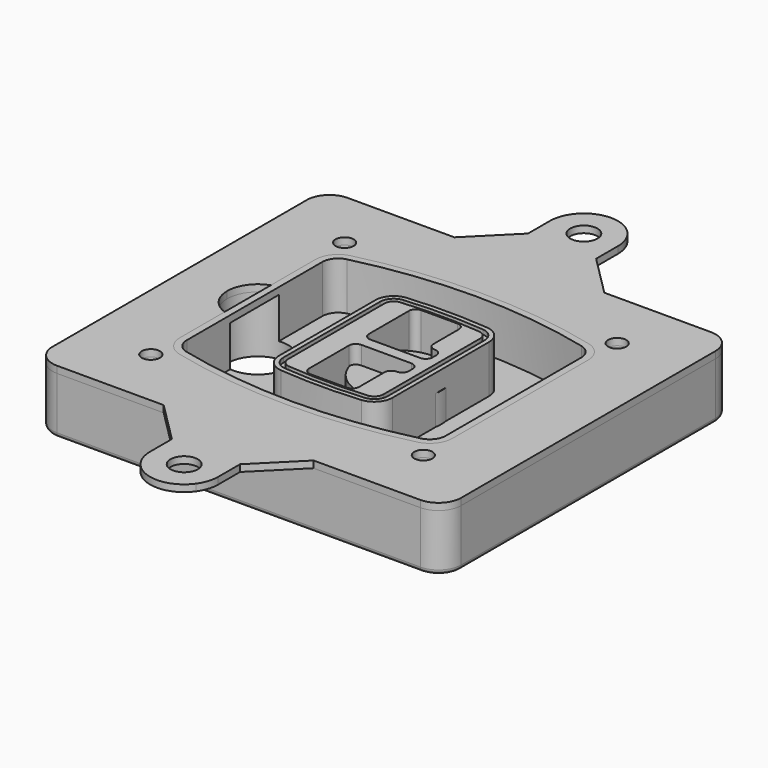
from build123d import *

# Parameters (mm, degrees)
F0_R      = 4
F1_DEPTH  = 25
F2_DEPTH  = 3
F3_DEPTH  = 18
F5_DEPTH  = 21
F6_DEPTH  = 2
F8_DEPTH  = 20
F9_DEPTH  = 16
F10_DEPTH = 25
F7_R      = 6
F7_R_2    = 4
F11_DEPTH = 6
F13_DEPTH = 9
F15_R     = 2
F16_R     = 6
F16_R_2   = 4
F17_DEPTH = 3


# Not quite as in the source:
# - a feature of the source that left no trace in its solid (it failed there, or was rolled back) is left out
# - a feature names something its author has since deleted; it is built from what else it names


with BuildPart() as f1:
    # F0 (on Top) → F1 (new body)
    with BuildSketch(Plane.XY):
        with BuildLine():
            ThreePointArc((-90, -70), (-87.0710678119, -77.0710678119), (-80, -80))
            Line((-80, -80), (80, -80))
            ThreePointArc((80, -80), (87.0710678119, -77.0710678119), (90, -70))
            Line((90, -70), (90, 70))
            ThreePointArc((90, 70), (87.0710678119, 77.0710678119), (80, 80))
            Line((80, 80), (-80, 80))
            ThreePointArc((-80, 80), (-87.0710678119, 77.0710678119), (-90, 70))
            Line((-90, 70), (-90, -70))
        make_face()
        with Locations((-60, -53.3333333333)):
            Circle(F0_R, mode=Mode.SUBTRACT)
        with Locations((60, -53.3333333333)):
            Circle(F0_R, mode=Mode.SUBTRACT)
        with Locations((-60, 53.3333333333)):
            Circle(F0_R, mode=Mode.SUBTRACT)
        with BuildLine():
            ThreePointArc((-64, 37.2990447398), (-61.0143011354, 45.9411029726), (-53.3306899286, 50.8970778549))
            ThreePointArc((-53.3306899286, 50.8970778549), (0, 57.3333333333), (53.3306899286, 50.8970778549))
            ThreePointArc((53.3306899286, 50.8970778549), (61.0143011354, 45.9411029726), (64, 37.2990447398))
            Line((64, 37.2990447398), (64, -37.2990447398))
            ThreePointArc((64, -37.2990447398), (61.0143011354, -45.9411029726), (53.3306899286, -50.8970778549))
            ThreePointArc((53.3306899286, -50.8970778549), (0, -57.3333333333), (-53.3306899286, -50.8970778549))
            ThreePointArc((-53.3306899286, -50.8970778549), (-61.0143011354, -45.9411029726), (-64, -37.2990447398))
            Line((-64, -37.2990447398), (-64, 37.2990447398))
        make_face(mode=Mode.SUBTRACT)
        with Locations((60, 53.3333333333)):
            Circle(F0_R, mode=Mode.SUBTRACT)
        with BuildLine():
            ThreePointArc((53.3306899286, 50.8970778549), (0, 57.3333333333), (-53.3306899286, 50.8970778549))
            ThreePointArc((-53.3306899286, 50.8970778549), (-61.0143011354, 45.9411029726), (-64, 37.2990447398))
            Line((-64, 37.2990447398), (-64, -37.2990447398))
            ThreePointArc((-64, -37.2990447398), (-61.0143011354, -45.9411029726), (-53.3306899286, -50.8970778549))
            ThreePointArc((-53.3306899286, -50.8970778549), (0, -57.3333333333), (53.3306899286, -50.8970778549))
            ThreePointArc((53.3306899286, -50.8970778549), (61.0143011354, -45.9411029726), (64, -37.2990447398))
            Line((64, -37.2990447398), (64, 37.2990447398))
            ThreePointArc((64, 37.2990447398), (61.0143011354, 45.9411029726), (53.3306899286, 50.8970778549))
        make_face()
        with BuildLine():
            Line((-60, -37.2990447398), (-60, 37.2990447398))
            ThreePointArc((-60, 37.2990447398), (-57.8673579538, 43.4719434775), (-52.3790642347, 47.0119255363))
            ThreePointArc((-52.3790642347, 47.0119255363), (0, 53.3333333333), (52.3790642347, 47.0119255363))
            ThreePointArc((52.3790642347, 47.0119255363), (57.8673579538, 43.4719434775), (60, 37.2990447398))
            Line((60, 37.2990447398), (60, -37.2990447398))
            ThreePointArc((60, -37.2990447398), (57.8673579538, -43.4719434775), (52.3790642347, -47.0119255363))
            ThreePointArc((52.3790642347, -47.0119255363), (0, -53.3333333333), (-52.3790642347, -47.0119255363))
            ThreePointArc((-52.3790642347, -47.0119255363), (-57.8673579538, -43.4719434775), (-60, -37.2990447398))
        make_face(mode=Mode.SUBTRACT)
        with BuildLine():
            ThreePointArc((-52.3790642347, 47.0119255363), (-57.8673579538, 43.4719434775), (-60, 37.2990447398))
            Line((-60, 37.2990447398), (-60, -37.2990447398))
            ThreePointArc((-60, -37.2990447398), (-57.8673579538, -43.4719434775), (-52.3790642347, -47.0119255363))
            ThreePointArc((-52.3790642347, -47.0119255363), (0, -53.3333333333), (52.3790642347, -47.0119255363))
            ThreePointArc((52.3790642347, -47.0119255363), (57.8673579538, -43.4719434775), (60, -37.2990447398))
            Line((60, -37.2990447398), (60, 37.2990447398))
            ThreePointArc((60, 37.2990447398), (57.8673579538, 43.4719434775), (52.3790642347, 47.0119255363))
            ThreePointArc((52.3790642347, 47.0119255363), (0, 53.3333333333), (-52.3790642347, 47.0119255363))
        make_face()
        with BuildLine():
            ThreePointArc((51.6653449643, 44.0980612973), (55.5071505677, 41.6200738562), (57, 37.2990447398))
            Line((57, 37.2990447398), (57, -37.2990447398))
            ThreePointArc((57, -37.2990447398), (55.5071505677, -41.6200738562), (51.6653449643, -44.0980612973))
            ThreePointArc((51.6653449643, -44.0980612973), (0, -50.3333333333), (-51.6653449643, -44.0980612973))
            ThreePointArc((-51.6653449643, -44.0980612973), (-55.5071505677, -41.6200738562), (-57, -37.2990447398))
            Line((-57, -37.2990447398), (-57, 37.2990447398))
            ThreePointArc((-57, 37.2990447398), (-55.5071505677, 41.6200738562), (-51.6653449643, 44.0980612973))
            ThreePointArc((-51.6653449643, 44.0980612973), (0, 50.3333333333), (51.6653449643, 44.0980612973))
        make_face(mode=Mode.SUBTRACT)
        with BuildLine():
            Line((57, -37.2990447398), (57, 37.2990447398))
            ThreePointArc((57, 37.2990447398), (55.5071505677, 41.6200738562), (51.6653449643, 44.0980612973))
            ThreePointArc((51.6653449643, 44.0980612973), (0, 50.3333333333), (-51.6653449643, 44.0980612973))
            ThreePointArc((-51.6653449643, 44.0980612973), (-55.5071505677, 41.6200738562), (-57, 37.2990447398))
            Line((-57, 37.2990447398), (-57, -37.2990447398))
            ThreePointArc((-57, -37.2990447398), (-55.5071505677, -41.6200738562), (-51.6653449643, -44.0980612973))
            ThreePointArc((-51.6653449643, -44.0980612973), (0, -50.3333333333), (51.6653449643, -44.0980612973))
            ThreePointArc((51.6653449643, -44.0980612973), (55.5071505677, -41.6200738562), (57, -37.2990447398))
        make_face()
    extrude(amount=-F1_DEPTH)

    # F0 (on Top) → F2 (join)
    with BuildSketch(Plane.XY):
        with BuildLine():
            ThreePointArc((-52.3790642347, 47.0119255363), (-57.8673579538, 43.4719434775), (-60, 37.2990447398))
            Line((-60, 37.2990447398), (-60, -37.2990447398))
            ThreePointArc((-60, -37.2990447398), (-57.8673579538, -43.4719434775), (-52.3790642347, -47.0119255363))
            ThreePointArc((-52.3790642347, -47.0119255363), (0, -53.3333333333), (52.3790642347, -47.0119255363))
            ThreePointArc((52.3790642347, -47.0119255363), (57.8673579538, -43.4719434775), (60, -37.2990447398))
            Line((60, -37.2990447398), (60, 37.2990447398))
            ThreePointArc((60, 37.2990447398), (57.8673579538, 43.4719434775), (52.3790642347, 47.0119255363))
            ThreePointArc((52.3790642347, 47.0119255363), (0, 53.3333333333), (-52.3790642347, 47.0119255363))
        make_face()
        with BuildLine():
            ThreePointArc((51.6653449643, 44.0980612973), (55.5071505677, 41.6200738562), (57, 37.2990447398))
            Line((57, 37.2990447398), (57, -37.2990447398))
            ThreePointArc((57, -37.2990447398), (55.5071505677, -41.6200738562), (51.6653449643, -44.0980612973))
            ThreePointArc((51.6653449643, -44.0980612973), (0, -50.3333333333), (-51.6653449643, -44.0980612973))
            ThreePointArc((-51.6653449643, -44.0980612973), (-55.5071505677, -41.6200738562), (-57, -37.2990447398))
            Line((-57, -37.2990447398), (-57, 37.2990447398))
            ThreePointArc((-57, 37.2990447398), (-55.5071505677, 41.6200738562), (-51.6653449643, 44.0980612973))
            ThreePointArc((-51.6653449643, 44.0980612973), (0, 50.3333333333), (51.6653449643, 44.0980612973))
        make_face(mode=Mode.SUBTRACT)
    extrude(amount=F2_DEPTH)

    # F0 (on Top) → F3 (cut)
    with BuildSketch(Plane.XY):
        with BuildLine():
            Line((57, -37.2990447398), (57, 37.2990447398))
            ThreePointArc((57, 37.2990447398), (55.5071505677, 41.6200738562), (51.6653449643, 44.0980612973))
            ThreePointArc((51.6653449643, 44.0980612973), (0, 50.3333333333), (-51.6653449643, 44.0980612973))
            ThreePointArc((-51.6653449643, 44.0980612973), (-55.5071505677, 41.6200738562), (-57, 37.2990447398))
            Line((-57, 37.2990447398), (-57, -37.2990447398))
            ThreePointArc((-57, -37.2990447398), (-55.5071505677, -41.6200738562), (-51.6653449643, -44.0980612973))
            ThreePointArc((-51.6653449643, -44.0980612973), (0, -50.3333333333), (51.6653449643, -44.0980612973))
            ThreePointArc((51.6653449643, -44.0980612973), (55.5071505677, -41.6200738562), (57, -37.2990447398))
        make_face()
    extrude(amount=-F3_DEPTH, mode=Mode.SUBTRACT)

    # F4 (on face) → F5 (join, through all)
    with BuildSketch(Plane.XY.offset(3)):
        with BuildLine():
            ThreePointArc((-25, -26.587695628), (-22.8992979869, -31.9912392117), (-17.7004291845, -34.5569740744))
            ThreePointArc((-17.7004291845, -34.5569740744), (0, -35.3333333333), (17.7004291845, -34.5569740744))
            ThreePointArc((17.7004291845, -34.5569740744), (22.8992979869, -31.9912392117), (25, -26.587695628))
            Line((25, -26.587695628), (25, 26.587695628))
            ThreePointArc((25, 26.587695628), (22.8992979869, 31.9912392117), (17.7004291845, 34.5569740744))
            ThreePointArc((17.7004291845, 34.5569740744), (0, 35.3333333333), (-17.7004291845, 34.5569740744))
            ThreePointArc((-17.7004291845, 34.5569740744), (-22.8992979869, 31.9912392117), (-25, 26.587695628))
            Line((-25, 26.587695628), (-25, -26.587695628))
        make_face()
        with BuildLine():
            ThreePointArc((17.5253218884, 32.5646544628), (21.4244734902, 30.6403533158), (23, 26.587695628))
            Line((23, 26.587695628), (23, -26.587695628))
            ThreePointArc((23, -26.587695628), (21.4244734902, -30.6403533158), (17.5253218884, -32.5646544628))
            ThreePointArc((17.5253218884, -32.5646544628), (0, -33.3333333333), (-17.5253218884, -32.5646544628))
            ThreePointArc((-17.5253218884, -32.5646544628), (-21.4244734902, -30.6403533158), (-23, -26.587695628))
            Line((-23, -26.587695628), (-23, 26.587695628))
            ThreePointArc((-23, 26.587695628), (-21.4244734902, 30.6403533158), (-17.5253218884, 32.5646544628))
            ThreePointArc((-17.5253218884, 32.5646544628), (0, 33.3333333333), (17.5253218884, 32.5646544628))
        make_face(mode=Mode.SUBTRACT)
        with BuildLine():
            Line((23, -26.587695628), (23, 26.587695628))
            ThreePointArc((23, 26.587695628), (21.4244734902, 30.6403533158), (17.5253218884, 32.5646544628))
            ThreePointArc((17.5253218884, 32.5646544628), (0, 33.3333333333), (-17.5253218884, 32.5646544628))
            ThreePointArc((-17.5253218884, 32.5646544628), (-21.4244734902, 30.6403533158), (-23, 26.587695628))
            Line((-23, 26.587695628), (-23, -26.587695628))
            ThreePointArc((-23, -26.587695628), (-21.4244734902, -30.6403533158), (-17.5253218884, -32.5646544628))
            ThreePointArc((-17.5253218884, -32.5646544628), (0, -33.3333333333), (17.5253218884, -32.5646544628))
            ThreePointArc((17.5253218884, -32.5646544628), (21.4244734902, -30.6403533158), (23, -26.587695628))
        make_face()
        with BuildLine():
            ThreePointArc((17.3502145923, 30.5723348512), (19.9496489934, 29.2894674198), (21, 26.587695628))
            Line((21, 26.587695628), (21, -26.587695628))
            ThreePointArc((21, -26.587695628), (19.9496489934, -29.2894674198), (17.3502145923, -30.5723348512))
            ThreePointArc((17.3502145923, -30.5723348512), (0, -31.3333333333), (-17.3502145923, -30.5723348512))
            ThreePointArc((-17.3502145923, -30.5723348512), (-19.9496489934, -29.2894674198), (-21, -26.587695628))
            Line((-21, -26.587695628), (-21, 26.587695628))
            ThreePointArc((-21, 26.587695628), (-19.9496489934, 29.2894674198), (-17.3502145923, 30.5723348512))
            ThreePointArc((-17.3502145923, 30.5723348512), (0, 31.3333333333), (17.3502145923, 30.5723348512))
        make_face(mode=Mode.SUBTRACT)
        with BuildLine():
            Line((21, -26.587695628), (21, 26.587695628))
            ThreePointArc((21, 26.587695628), (19.9496489934, 29.2894674198), (17.3502145923, 30.5723348512))
            ThreePointArc((17.3502145923, 30.5723348512), (0, 31.3333333333), (-17.3502145923, 30.5723348512))
            ThreePointArc((-17.3502145923, 30.5723348512), (-19.9496489934, 29.2894674198), (-21, 26.587695628))
            Line((-21, 26.587695628), (-21, -26.587695628))
            ThreePointArc((-21, -26.587695628), (-19.9496489934, -29.2894674198), (-17.3502145923, -30.5723348512))
            ThreePointArc((-17.3502145923, -30.5723348512), (0, -31.3333333333), (17.3502145923, -30.5723348512))
            ThreePointArc((17.3502145923, -30.5723348512), (19.9496489934, -29.2894674198), (21, -26.587695628))
        make_face()
        with BuildLine():
            Line((-8, -2.5), (14, -2.5))
            ThreePointArc((14, -2.5), (16.1213203436, -3.3786796564), (17, -5.5))
            Line((17, -5.5), (17, -7.5))
            ThreePointArc((17, -7.5), (16.1213203436, -9.6213203436), (14, -10.5))
            ThreePointArc((14, -10.5), (11.8786796564, -11.3786796564), (11, -13.5))
            Line((11, -13.5), (11, -27.5))
            ThreePointArc((11, -27.5), (10.1213203436, -29.6213203436), (8, -30.5))
            Line((8, -30.5), (-8, -30.5))
            ThreePointArc((-8, -30.5), (-10.1213203436, -29.6213203436), (-11, -27.5))
            Line((-11, -27.5), (-11, -5.5))
            ThreePointArc((-11, -5.5), (-10.1213203436, -3.3786796564), (-8, -2.5))
        make_face(mode=Mode.SUBTRACT)
        with BuildLine():
            ThreePointArc((-8, 2.5), (-10.1213203436, 3.3786796564), (-11, 5.5))
            Line((-11, 5.5), (-11, 27.5))
            ThreePointArc((-11, 27.5), (-10.1213203436, 29.6213203436), (-8, 30.5))
            Line((-8, 30.5), (8, 30.5))
            ThreePointArc((8, 30.5), (10.1213203436, 29.6213203436), (11, 27.5))
            Line((11, 27.5), (11, 13.5))
            ThreePointArc((11, 13.5), (11.8786796564, 11.3786796564), (14, 10.5))
            ThreePointArc((14, 10.5), (16.1213203436, 9.6213203436), (17, 7.5))
            Line((17, 7.5), (17, 5.5))
            ThreePointArc((17, 5.5), (16.1213203436, 3.3786796564), (14, 2.5))
            Line((14, 2.5), (-8, 2.5))
        make_face(mode=Mode.SUBTRACT)
    extrude(amount=-F5_DEPTH)

    # F4 (on face) → F6 (cut)
    with BuildSketch(Plane.XY.offset(3)):
        with BuildLine():
            Line((23, -26.587695628), (23, 26.587695628))
            ThreePointArc((23, 26.587695628), (21.4244734902, 30.6403533158), (17.5253218884, 32.5646544628))
            ThreePointArc((17.5253218884, 32.5646544628), (0, 33.3333333333), (-17.5253218884, 32.5646544628))
            ThreePointArc((-17.5253218884, 32.5646544628), (-21.4244734902, 30.6403533158), (-23, 26.587695628))
            Line((-23, 26.587695628), (-23, -26.587695628))
            ThreePointArc((-23, -26.587695628), (-21.4244734902, -30.6403533158), (-17.5253218884, -32.5646544628))
            ThreePointArc((-17.5253218884, -32.5646544628), (0, -33.3333333333), (17.5253218884, -32.5646544628))
            ThreePointArc((17.5253218884, -32.5646544628), (21.4244734902, -30.6403533158), (23, -26.587695628))
        make_face()
        with BuildLine():
            ThreePointArc((17.3502145923, 30.5723348512), (19.9496489934, 29.2894674198), (21, 26.587695628))
            Line((21, 26.587695628), (21, -26.587695628))
            ThreePointArc((21, -26.587695628), (19.9496489934, -29.2894674198), (17.3502145923, -30.5723348512))
            ThreePointArc((17.3502145923, -30.5723348512), (0, -31.3333333333), (-17.3502145923, -30.5723348512))
            ThreePointArc((-17.3502145923, -30.5723348512), (-19.9496489934, -29.2894674198), (-21, -26.587695628))
            Line((-21, -26.587695628), (-21, 26.587695628))
            ThreePointArc((-21, 26.587695628), (-19.9496489934, 29.2894674198), (-17.3502145923, 30.5723348512))
            ThreePointArc((-17.3502145923, 30.5723348512), (0, 31.3333333333), (17.3502145923, 30.5723348512))
        make_face(mode=Mode.SUBTRACT)
    extrude(amount=-F6_DEPTH, mode=Mode.SUBTRACT)

    # F7 (on face) → F8 (join)
    with BuildSketch(Plane(origin=(0, 0, -25), x_dir=(1, 0, 0), z_dir=(0, 0, -1))):
        with BuildLine():
            ThreePointArc((-6.71157564, 0), (6.7567035675, 13.4682792075), (20.224982775, 0))
            Line((20.224982775, 0), (25.224982775, 0))
            ThreePointArc((25.224982775, 0), (6.7567035675, 18.4682792075), (-11.71157564, 0))
            Line((-11.71157564, 0), (-6.71157564, 0))
        make_face()
        with BuildLine():
            Line((-6.71157564, 0), (20.224982775, 0))
            ThreePointArc((20.224982775, 0), (6.7567035675, 13.4682792075), (-6.71157564, 0))
        make_face()
        with BuildLine():
            ThreePointArc((-6.71157564, 0), (6.7567035675, -13.4682792075), (20.224982775, 0))
            Line((20.224982775, 0), (-6.71157564, 0))
        make_face()
        with BuildLine():
            Line((25.224982775, 0), (20.224982775, 0))
            ThreePointArc((20.224982775, 0), (6.7567035675, -13.4682792075), (-6.71157564, 0))
            Line((-6.71157564, 0), (-11.71157564, 0))
            ThreePointArc((-11.71157564, 0), (6.7567035675, -18.4682792075), (25.224982775, 0))
        make_face()
    extrude(amount=-F8_DEPTH)

    # F7 (on face) → F9 (cut)
    with BuildSketch(Plane(origin=(0, 0, -25), x_dir=(1, 0, 0), z_dir=(0, 0, -1))):
        with BuildLine():
            Line((-6.71157564, 0), (20.224982775, 0))
            ThreePointArc((20.224982775, 0), (6.7567035675, 13.4682792075), (-6.71157564, 0))
        make_face()
        with BuildLine():
            ThreePointArc((-6.71157564, 0), (6.7567035675, -13.4682792075), (20.224982775, 0))
            Line((20.224982775, 0), (-6.71157564, 0))
        make_face()
    extrude(amount=-F9_DEPTH, mode=Mode.SUBTRACT)

    # F7 (on face) → F10 (cut)
    with BuildSketch(Plane(origin=(0, 0, -25), x_dir=(1, 0, 0), z_dir=(0, 0, -1))):
        with BuildLine():
            Line((-69.0318229325, 0), (-42.0952645175, 0))
            ThreePointArc((-42.0952645175, 0), (-55.563543725, 13.4682792075), (-69.0318229325, 0))
        make_face()
        with BuildLine():
            ThreePointArc((-69.0318229325, 0), (-55.563543725, -13.4682792075), (-42.0952645175, 0))
            Line((-42.0952645175, 0), (-69.0318229325, 0))
        make_face()
    extrude(amount=-F10_DEPTH, mode=Mode.SUBTRACT)

    # F7 (on face) → F11 (cut)
    with BuildSketch(Plane(origin=(0, 0, -25), x_dir=(1, 0, 0), z_dir=(0, 0, -1))):
        with Locations((60, -53.3333333333)):
            Circle(F7_R)
        with Locations((60, -53.3333333333)):
            Circle(F7_R_2, mode=Mode.SUBTRACT)
        with Locations((-60, -53.3333333333)):
            Circle(F7_R)
        with Locations((-60, -53.3333333333)):
            Circle(F7_R_2, mode=Mode.SUBTRACT)
        with Locations((-60, 53.3333333333)):
            Circle(F7_R)
        with Locations((-60, 53.3333333333)):
            Circle(F7_R_2, mode=Mode.SUBTRACT)
        with Locations((60, 53.3333333333)):
            Circle(F7_R)
        with Locations((60, 53.3333333333)):
            Circle(F7_R_2, mode=Mode.SUBTRACT)
    extrude(amount=-F11_DEPTH, mode=Mode.SUBTRACT)

    # F12 (on face) → F13 (cut, through all)
    with BuildSketch(Plane(origin=(0, 0, -9), x_dir=(1, 0, 0), z_dir=(0, 0, -1))):
        with BuildLine():
            ThreePointArc((20.224982775, 0), (20.1663399806, 1.2554664788), (19.9909222755, 2.5))
            Line((19.9909222755, 2.5), (14, 2.5))
            ThreePointArc((14, 2.5), (16.1213203436, 3.3786796564), (17, 5.5))
            Line((17, 5.5), (17, 7.5))
            ThreePointArc((17, 7.5), (16.1213203436, 9.6213203436), (14, 10.5))
            ThreePointArc((14, 10.5), (12.1627255951, 11.1284134507), (11.0951631559, 12.750384826))
            ThreePointArc((11.0951631559, 12.750384826), (11.0476113807, 12.7664660322), (11, 12.7823698976))
            Line((11, 12.7823698976), (11, -12.7823698976))
            ThreePointArc((11, -12.7823698976), (11.0476113807, -12.7664660322), (11.0951631559, -12.750384826))
            ThreePointArc((11.0951631559, -12.750384826), (12.1627255951, -11.1284134507), (14, -10.5))
            ThreePointArc((14, -10.5), (16.1213203436, -9.6213203436), (17, -7.5))
            Line((17, -7.5), (17, -5.5))
            ThreePointArc((17, -5.5), (16.1213203436, -3.3786796564), (14, -2.5))
            Line((14, -2.5), (19.9909222755, -2.5))
            ThreePointArc((19.9909222755, -2.5), (20.1663399806, -1.2554664788), (20.224982775, 0))
        make_face()
    extrude(amount=F13_DEPTH, mode=Mode.SUBTRACT)

    # F15
    f15_edges = [f1.edges().sort_by_distance(p)[0] for p in [
        (0, -80, -25),
        (-87.071068, -77.071068, -25),
        (-90, 0, -25),
        (-87.071068, 77.071068, -25),
        (87.071068, -77.071068, -25),
        (0, 80, -25),
        (90, 0, -25),
        (87.071068, 77.071068, -25),
    ]]
    fillet(f15_edges, radius=F15_R)


with BuildPart() as f17:
    # F16 (on face) → F17 (new body, through all)
    with BuildSketch(Plane.XY):
        with BuildLine():
            ThreePointArc((15, 110), (14.2918775795, 114.5543644179), (12.2343686332, 118.6787224952))
            ThreePointArc((12.2343686332, 118.6787224952), (0, 125), (-12.2343686332, 118.6787224952))
            ThreePointArc((-12.2343686332, 118.6787224952), (-14.2918775795, 114.5543644179), (-15, 110))
            Line((-15, 110), (-15, 98))
            Line((-15, 98), (-33, 80))
            Line((-33, 80), (33, 80))
            Line((33, 80), (15, 98))
            Line((15, 98), (15, 110))
        make_face()
        with Locations((0, 110)):
            Circle(F16_R, mode=Mode.SUBTRACT)
        with BuildLine():
            Line((80, 80), (33, 80))
            Line((33, 80), (-33, 80))
            Line((-33, 80), (-80, 80))
            ThreePointArc((-80, 80), (-87.0710678119, 77.0710678119), (-90, 70))
            Line((-90, 70), (-90, -70))
            ThreePointArc((-90, -70), (-87.0710678119, -77.0710678119), (-80, -80))
            Line((-80, -80), (-33, -80))
            Line((-33, -80), (33, -80))
            Line((33, -80), (80, -80))
            ThreePointArc((80, -80), (87.0710678119, -77.0710678119), (90, -70))
            Line((90, -70), (90, 70))
            ThreePointArc((90, 70), (87.0710678119, 77.0710678119), (80, 80))
        make_face()
        with Locations((-60, -53.3333333333)):
            Circle(F16_R_2, mode=Mode.SUBTRACT)
        with BuildLine():
            ThreePointArc((-60, 37.2990447398), (-57.8673579538, 43.4719434775), (-52.3790642347, 47.0119255363))
            ThreePointArc((-52.3790642347, 47.0119255363), (0, 53.3333333333), (52.3790642347, 47.0119255363))
            ThreePointArc((52.3790642347, 47.0119255363), (57.8673579538, 43.4719434775), (60, 37.2990447398))
            Line((60, 37.2990447398), (60, -37.2990447398))
            ThreePointArc((60, -37.2990447398), (57.8673579538, -43.4719434775), (52.3790642347, -47.0119255363))
            ThreePointArc((52.3790642347, -47.0119255363), (0, -53.3333333333), (-52.3790642347, -47.0119255363))
            ThreePointArc((-52.3790642347, -47.0119255363), (-57.8673579538, -43.4719434775), (-60, -37.2990447398))
            Line((-60, -37.2990447398), (-60, -12.7166190685))
            ThreePointArc((-60, -12.7166190685), (-66.5441169481, -7.798817635), (-69.0318229325, 0))
            ThreePointArc((-69.0318229325, 0), (-66.5441169481, 7.798817635), (-60, 12.7166190685))
            Line((-60, 12.7166190685), (-60, 37.2990447398))
        make_face(mode=Mode.SUBTRACT)
        with Locations((60, -53.3333333333)):
            Circle(F16_R_2, mode=Mode.SUBTRACT)
        with Locations((-60, 53.3333333333)):
            Circle(F16_R_2, mode=Mode.SUBTRACT)
        with Locations((60, 53.3333333333)):
            Circle(F16_R_2, mode=Mode.SUBTRACT)
        with BuildLine():
            Line((15, -98), (33, -80))
            Line((33, -80), (-33, -80))
            Line((-33, -80), (-15, -98))
            Line((-15, -98), (-15, -110))
            ThreePointArc((-15, -110), (-14.2918775795, -114.5543644179), (-12.2343686332, -118.6787224952))
            ThreePointArc((-12.2343686332, -118.6787224952), (0, -125), (12.2343686332, -118.6787224952))
            ThreePointArc((12.2343686332, -118.6787224952), (14.2918775795, -114.5543644179), (15, -110))
            Line((15, -110), (15, -98))
        make_face()
        with Locations((0, -110)):
            Circle(F16_R, mode=Mode.SUBTRACT)
    extrude(amount=F17_DEPTH)


solid = Compound([f1.part, f17.part])
